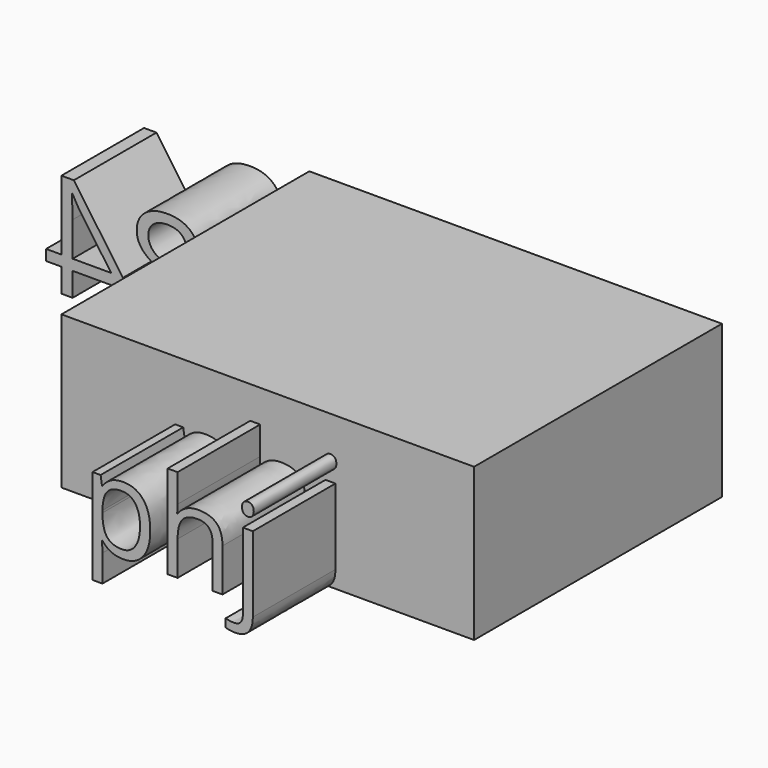
from build123d import *

# Parameters (mm, degrees)
F0_W         = 101.4873385429
F0_H         = 37.5162102282
F1_DEPTH     = 50.8
F3_TEXT_SIZE = 35.6009242953
F4_DEPTH     = 25.4
F2_TEXT_SIZE = 30.1434244547
F5_DEPTH     = 25.4


# Not quite as in the source:
# - Text() gives the source's letters only with a copy of the font that has no kerning and outlines rounded to 1/6400 em; it was checked with that copy


with BuildPart() as f1:
    # F0 (on Front) → F1 (new body)
    with BuildSketch(Plane.XZ):
        with Locations((50.7436692715, 18.7581051141)):
            Rectangle(F0_W, F0_H)
    extrude(amount=F1_DEPTH)

    # F3 (on face) → F4 (join)
    with BuildSketch(Plane(origin=(0, 0, 0), x_dir=(-1, 0, 0), z_dir=(0, 1, 0))):
        Polygon((0, 0), (0, 13.9621879583), (-0.0585577086, 13.9621879583), (-0.0585577086, 8.1214113161), (-2.823191986, 8.1214113161), (-2.823191986, 13.9621879583), (-15.1833878897, 13.9621879583), (-15.1833878897, 16.4820658811), (-3.1180121403, 33.6761997868), (-0.0585577086, 33.6761997868), (-0.0585577086, 16.5877561251), (0, 16.5877561251), (0, 37.5162102282), (-101.4873385429, 37.5162102282), (-101.4873385429, 0), align=None)
        with BuildLine():
            add(Edge.make_bspline(
                [(-80.9060317254, 30.5805881664), (-78.7588509789, 27.2235322583), (-78.7588509789, 20.8654296849)],
                knots=[0, 0, 0, 1, 1, 1], degree=2))
            add(Edge.make_bspline(
                [(-78.7588509789, 20.8654296849), (-78.7588509789, 14.2736960459), (-80.8364986702, 11.0223303817)],
                knots=[0, 0, 0, 1, 1, 1], degree=2))
            add(Edge.make_bspline(
                [(-80.8364986702, 11.0223303817), (-82.9141463615, 7.7709647176), (-87.1918199213, 7.7709647176)],
                knots=[0, 0, 0, 1, 1, 1], degree=2))
            add(Edge.make_bspline(
                [(-87.1918199213, 7.7709647176), (-91.2914888597, 7.7709647176), (-93.4303256396, 11.1002074036)],
                knots=[0, 0, 0, 1, 1, 1], degree=2))
            add(Edge.make_bspline(
                [(-93.4303256396, 11.1002074036), (-95.5691624196, 14.4294500897), (-95.5691624196, 20.8654296849)],
                knots=[0, 0, 0, 1, 1, 1], degree=2))
            add(Edge.make_bspline(
                [(-95.5691624196, 20.8654296849), (-95.5691624196, 27.5016644793), (-93.4998586949, 30.719654277)],
                knots=[0, 0, 0, 1, 1, 1], degree=2))
            add(Edge.make_bspline(
                [(-93.4998586949, 30.719654277), (-91.4305549702, 33.9376440746), (-87.1918199213, 33.9376440746)],
                knots=[0, 0, 0, 1, 1, 1], degree=2))
            add(Edge.make_bspline(
                [(-87.1918199213, 33.9376440746), (-83.053212472, 33.9376440746), (-80.9060317254, 30.5805881664)],
                knots=[0, 0, 0, 1, 1, 1], degree=2))
        make_face(mode=Mode.SUBTRACT)
        with BuildLine():
            Line((-64.5629824161, 33.5371336763), (-64.5629824161, 8.1214113161))
            Line((-64.5629824161, 8.1214113161), (-67.3776804932, 8.1214113161))
            Line((-67.3776804932, 8.1214113161), (-67.3776804932, 26.2333815513))
            add(Edge.make_bspline(
                [(-67.3776804932, 26.2333815513), (-67.3776804932, 28.4973778307), (-67.2386143827, 30.5110551112)],
                knots=[0, 0, 0, 1, 1, 1], degree=2))
            add(Edge.make_bspline(
                [(-67.2386143827, 30.5110551112), (-67.6001862701, 30.1439205794), (-68.0535417904, 29.7461915033)],
                knots=[0, 0, 0, 1, 1, 1], degree=2))
            add(Edge.make_bspline(
                [(-68.0535417904, 29.7461915033), (-68.5068973107, 29.3484624272), (-72.1893679175, 26.3557597286)],
                knots=[0, 0, 0, 1, 1, 1], degree=2))
            Line((-72.1893679175, 26.3557597286), (-73.7190951333, 28.3360611425))
            Line((-73.7190951333, 28.3360611425), (-66.9938580282, 33.5371336763))
            Line((-66.9938580282, 33.5371336763), (-64.5629824161, 33.5371336763))
        make_face(mode=Mode.SUBTRACT)
        with BuildLine():
            add(Edge.make_bspline(
                [(-40.1985998516, 30.5805881664), (-38.051419105, 27.2235322583), (-38.051419105, 20.8654296849)],
                knots=[0, 0, 0, 1, 1, 1], degree=2))
            add(Edge.make_bspline(
                [(-38.051419105, 20.8654296849), (-38.051419105, 14.2736960459), (-40.1290667963, 11.0223303817)],
                knots=[0, 0, 0, 1, 1, 1], degree=2))
            add(Edge.make_bspline(
                [(-40.1290667963, 11.0223303817), (-42.2067144876, 7.7709647176), (-46.4843880474, 7.7709647176)],
                knots=[0, 0, 0, 1, 1, 1], degree=2))
            add(Edge.make_bspline(
                [(-46.4843880474, 7.7709647176), (-50.5840569858, 7.7709647176), (-52.7228937658, 11.1002074036)],
                knots=[0, 0, 0, 1, 1, 1], degree=2))
            add(Edge.make_bspline(
                [(-52.7228937658, 11.1002074036), (-54.8617305457, 14.4294500897), (-54.8617305457, 20.8654296849)],
                knots=[0, 0, 0, 1, 1, 1], degree=2))
            add(Edge.make_bspline(
                [(-54.8617305457, 20.8654296849), (-54.8617305457, 27.5016644793), (-52.792426821, 30.719654277)],
                knots=[0, 0, 0, 1, 1, 1], degree=2))
            add(Edge.make_bspline(
                [(-52.792426821, 30.719654277), (-50.7231230964, 33.9376440746), (-46.4843880474, 33.9376440746)],
                knots=[0, 0, 0, 1, 1, 1], degree=2))
            add(Edge.make_bspline(
                [(-46.4843880474, 33.9376440746), (-42.3457805981, 33.9376440746), (-40.1985998516, 30.5805881664)],
                knots=[0, 0, 0, 1, 1, 1], degree=2))
        make_face(mode=Mode.SUBTRACT)
        with BuildLine():
            add(Edge.make_bspline(
                [(-31.935291564, 10.735854194), (-34.246570321, 13.7007436705), (-34.246570321, 18.9852558706)],
                knots=[0, 0, 0, 1, 1, 1], degree=2))
            add(Edge.make_bspline(
                [(-34.246570321, 18.9852558706), (-34.246570321, 26.4781379058), (-31.3345259665, 30.1884217347)],
                knots=[0, 0, 0, 1, 1, 1], degree=2))
            add(Edge.make_bspline(
                [(-31.3345259665, 30.1884217347), (-28.422481612, 33.8987055636), (-22.7207710804, 33.8987055636)],
                knots=[0, 0, 0, 1, 1, 1], degree=2))
            add(Edge.make_bspline(
                [(-22.7207710804, 33.8987055636), (-20.7571575997, 33.8987055636), (-19.6279407822, 33.5705095428)],
                knots=[0, 0, 0, 1, 1, 1], degree=2))
            Line((-19.6279407822, 33.5705095428), (-19.6279407822, 31.0840074865))
            add(Edge.make_bspline(
                [(-19.6279407822, 31.0840074865), (-20.9685380877, 31.5178937514), (-22.6873952138, 31.5178937514)],
                knots=[0, 0, 0, 1, 1, 1], degree=2))
            add(Edge.make_bspline(
                [(-22.6873952138, 31.5178937514), (-26.7759388634, 31.5178937514), (-28.9314635766, 28.9729839287)],
                knots=[0, 0, 0, 1, 1, 1], degree=2))
            add(Edge.make_bspline(
                [(-28.9314635766, 28.9729839287), (-31.0869882897, 26.4280741061), (-31.2928061333, 20.9655572845)],
                knots=[0, 0, 0, 1, 1, 1], degree=2))
            Line((-31.2928061333, 20.9655572845), (-31.0869882897, 20.9655572845))
            add(Edge.make_bspline(
                [(-31.0869882897, 20.9655572845), (-29.1734386089, 23.9582599831), (-25.0348311595, 23.9582599831)],
                knots=[0, 0, 0, 1, 1, 1], degree=2))
            add(Edge.make_bspline(
                [(-25.0348311595, 23.9582599831), (-21.6082421961, 23.9582599831), (-19.6362847488, 21.8889562584)],
                knots=[0, 0, 0, 1, 1, 1], degree=2))
            add(Edge.make_bspline(
                [(-19.6362847488, 21.8889562584), (-17.6643273015, 19.8196525337), (-17.6643273015, 16.2762480375)],
                knots=[0, 0, 0, 1, 1, 1], degree=2))
            add(Edge.make_bspline(
                [(-17.6643273015, 16.2762480375), (-17.6643273015, 12.3100825652), (-19.8281959814, 10.0405236414)],
                knots=[0, 0, 0, 1, 1, 1], degree=2))
            add(Edge.make_bspline(
                [(-19.8281959814, 10.0405236414), (-21.9920646612, 7.7709647176), (-25.6800979124, 7.7709647176)],
                knots=[0, 0, 0, 1, 1, 1], degree=2))
            add(Edge.make_bspline(
                [(-25.6800979124, 7.7709647176), (-29.624012807, 7.7709647176), (-31.935291564, 10.735854194)],
                knots=[0, 0, 0, 1, 1, 1], degree=2))
        make_face(mode=Mode.SUBTRACT)
        with Locations((-97.3436459899, 8.1214113161)):
            Text('0106484', F3_TEXT_SIZE, font='Open Sans', text_align=(TextAlign.LEFT, TextAlign.BOTTOM))
    extrude(amount=F4_DEPTH)

    # F2 (on face) → F5 (join)
    with BuildSketch(Plane.XZ.offset(50.8)):
        with Locations((25.3762882203, 6.66552037)):
            Text('phj', F2_TEXT_SIZE, font='Open Sans', text_align=(TextAlign.LEFT, TextAlign.BOTTOM))
    extrude(amount=F5_DEPTH)


solid = f1.part
